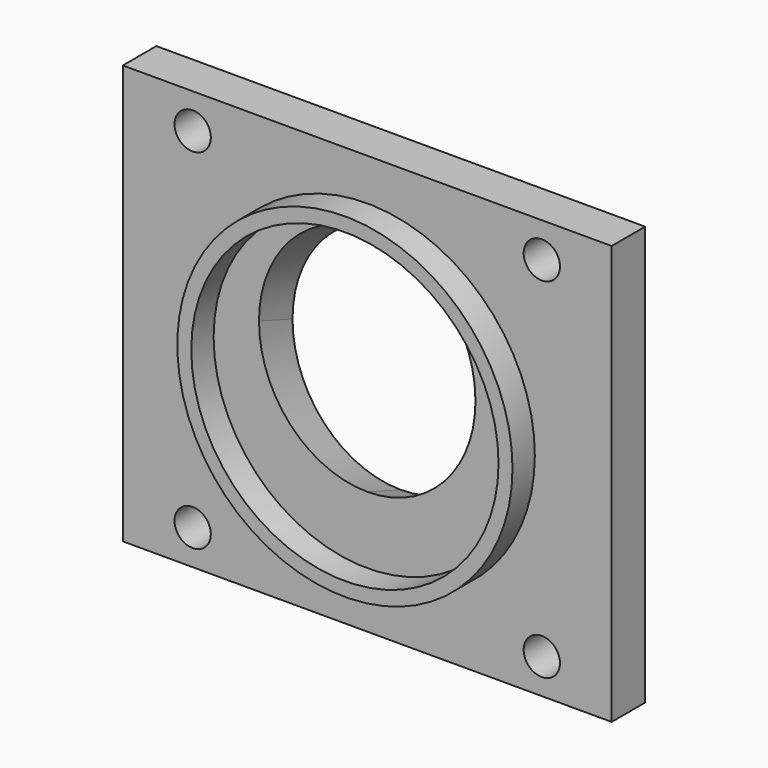
from build123d import *

# Parameters (mm, degrees)
F0_W     = 35
F0_H     = 30
F0_R     = 1.3
F0_R_2   = 12
F0_R_3   = 11
F1_DEPTH = 3
F3_DEPTH = 7.75
F4_R     = 7.74999
F5_DEPTH = 5


# Not quite as in the source:
# - a fillet or chamfer is up to 0.001 mm smaller than in the source, because OpenCascade refuses the exact size


with BuildPart() as f1:
    # F0 (on Front) → F1 (new body)
    with BuildSketch(Plane.XZ):
        Rectangle(F0_W, F0_H)
        with Locations((-12.5, -12.5)):
            Circle(F0_R, mode=Mode.SUBTRACT)
        with Locations((12.5, -12.5)):
            Circle(F0_R, mode=Mode.SUBTRACT)
        with Locations((-12.5, 12.5)):
            Circle(F0_R, mode=Mode.SUBTRACT)
        Circle(F0_R_2, mode=Mode.SUBTRACT)
        with Locations((12.5, 12.5)):
            Circle(F0_R, mode=Mode.SUBTRACT)
        Circle(F0_R_2)
        Circle(F0_R_3, mode=Mode.SUBTRACT)
        Circle(F0_R_3)
    extrude(amount=F1_DEPTH)

    # F2 (on Right) → F3 (cut, symmetric)
    with BuildSketch(Plane.YZ):
        Polygon((24.7599773954, -16.2912994583), (30.0612896169, -1.7260638362), (-14.6986877785, 14.5652356222), (-20, 0), align=None)
    extrude(amount=F3_DEPTH, both=True, mode=Mode.SUBTRACT)

    # F4 (radius 7.75 in the source; OpenCascade refuses exactly that, so slightly less here)
    f4_edges = [f1.edges().sort_by_distance(p)[0] for p in [
        (7.75, -1.5, 9.761306),
        (-7.75, -1.5, 9.761306),
        (-7.75, -1.5, -6.733449),
        (7.75, -1.5, -6.733449),
    ]]
    fillet(f4_edges, radius=F4_R)

    # F0 (on Front) → F5 (join)
    with BuildSketch(Plane.XZ):
        Circle(F0_R_2)
        Circle(F0_R_3, mode=Mode.SUBTRACT)
    extrude(amount=F5_DEPTH)


solid = f1.part
